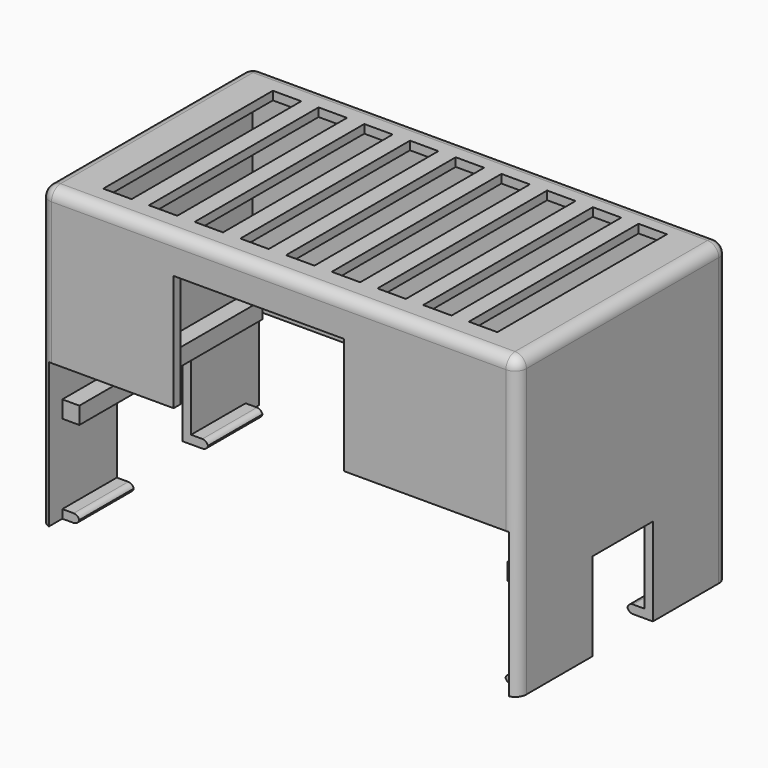
from build123d import *

# Parameters (mm, degrees)
F0_W         = 84
F0_H         = 46.33
F1_DEPTH     = 37
F2_T         = -1.5
F4_W         = 81
F4_H         = 10
F5_DEPTH     = 1.5
F6_W         = 30
F6_H         = 20.5
F7_DEPTH     = 1.5
F9_DEPTH     = 15.5
F10_W        = 40.33
F10_H        = 3
F11_DEPTH    = 3
F12_W        = 39.33
F12_H        = 3
F13_DEPTH    = 3
F14_W        = 1.5
F14_H        = 13.33
F15_DEPTH    = 15.5
F16_W        = 1.5
F16_H        = 16.33
F17_DEPTH    = 15.5
F18_W        = 12
F18_H        = 1.5
F19_DEPTH    = 3
F20_W        = 13.5
F20_H        = 1.5
F21_DEPTH    = 3
F22_W        = 5
F22_H        = 37.33
F23_DEPTH    = 1.5
F24_R        = 2
F25_T1_DEPTH = 17
F25_T3_DEPTH = 17
F25_T5_DEPTH = 18.5
F25_T7_DEPTH = 18.5


# Not quite as in the source:
# - a fillet or chamfer that OpenCascade refuses, or shapes differently, is made with other operations: its cross-section is extruded or revolved along the edge and cut away or added


with BuildPart() as f1:
    # F0 (on Top) → F1 (new body)
    with BuildSketch(Plane.XY):
        with Locations((42, 23.165)):
            Rectangle(F0_W, F0_H)
    extrude(amount=-F1_DEPTH)

    # F2
    f2_openings = [f1.faces().sort_by_distance(p)[0] for p in [
        (42, 23.165, -37),
    ]]
    offset(amount=F2_T, openings=f2_openings)

    # F4 (on face) → F5 (cut, through all)
    with BuildSketch(Plane.XZ):
        with Locations((42, -32)):
            Rectangle(F4_W, F4_H)
    extrude(amount=-F5_DEPTH, mode=Mode.SUBTRACT)

    # F6 (on face) → F7 (cut, through all)
    with BuildSketch(Plane.XZ):
        with Locations((38.5, -16.75)):
            Rectangle(F6_W, F6_H)
    extrude(amount=-F7_DEPTH, mode=Mode.SUBTRACT)

    # F8 (on face) → F9 (join)
    with BuildSketch(Plane(origin=(0, 0, -37), x_dir=(1, 0, 0), z_dir=(0, 0, -1))):
        Polygon((0, 0), (0, -46.33), (1.5, -46.33), (1.5, -44.83), (1.5, 0), align=None)
        Polygon((82.5, -44.83), (82.5, -46.33), (84, -46.33), (84, 0), (82.5, 0), align=None)
    extrude(amount=F9_DEPTH)

    # F10 (on face) → F11 (join)
    with BuildSketch(Plane.YZ.offset(1.5)):
        with Locations((23.165, -35.5)):
            Rectangle(F10_W, F10_H)
    extrude(amount=F11_DEPTH)

    # F12 (on face) → F13 (join)
    with BuildSketch(Plane(origin=(82.5, 0, 0), x_dir=(0, -1, 0), z_dir=(-1, 0, 0))):
        with Locations((-23.165, -35.5)):
            Rectangle(F12_W, F12_H)
    extrude(amount=F13_DEPTH)

    # F14 (on face) → F15 (cut)
    with BuildSketch(Plane(origin=(0, 0, -52.5), x_dir=(1, 0, 0), z_dir=(0, 0, -1))):
        with Locations((83.25, -23.165)):
            Rectangle(F14_W, F14_H)
    extrude(amount=-F15_DEPTH, mode=Mode.SUBTRACT)

    # F16 (on face) → F17 (cut)
    with BuildSketch(Plane(origin=(0, 0, -52.5), x_dir=(1, 0, 0), z_dir=(0, 0, -1))):
        with Locations((0.75, -23.165)):
            Rectangle(F16_W, F16_H)
    extrude(amount=-F17_DEPTH, mode=Mode.SUBTRACT)

    # F18 (on face) → F19 (join)
    with BuildSketch(Plane.YZ.offset(1.5)):
        with Locations((37.33, -51.75)):
            Rectangle(F18_W, F18_H)
        with Locations((9, -51.75)):
            Rectangle(F18_W, F18_H)
    extrude(amount=F19_DEPTH)

    # F20 (on face) → F21 (join)
    with BuildSketch(Plane(origin=(82.5, 0, 0), x_dir=(0, -1, 0), z_dir=(-1, 0, 0))):
        with Locations((-9.75, -51.75)):
            Rectangle(F20_W, F20_H)
        with Locations((-36.58, -51.75)):
            Rectangle(F20_W, F20_H)
    extrude(amount=F21_DEPTH)

    # F22 (on face) → F23 (cut, through all)
    with BuildSketch(Plane(origin=(0, 0, -1.5), x_dir=(1, 0, 0), z_dir=(0, 0, -1))):
        with Locations((73.9982255152, -23.6415825304)):
            Rectangle(F22_W, F22_H)
        with Locations((65.9984473258, -23.5820097141)):
            Rectangle(F22_W, F22_H)
        with Locations((49.998890947, -23.4628640815)):
            Rectangle(F22_W, F22_H)
        with Locations((41.9991127576, -23.4032912652)):
            Rectangle(F22_W, F22_H)
        with Locations((33.9993345682, -23.3437184489)):
            Rectangle(F22_W, F22_H)
        with Locations((25.9995563788, -23.2841456326)):
            Rectangle(F22_W, F22_H)
        with Locations((17.9997781894, -23.2245728163)):
            Rectangle(F22_W, F22_H)
        with Locations((10, -23.165)):
            Rectangle(F22_W, F22_H)
        with Locations((57.9986691364, -23.5224368978)):
            Rectangle(F22_W, F22_H)
    extrude(amount=-F23_DEPTH, mode=Mode.SUBTRACT)

    # F24
    f24_edges = [f1.edges().sort_by_distance(p)[0] for p in [
        (42, 0, 0),
        (84, 23.165, 0),
        (84, 0, -26.25),
        (84, 46.33, -26.25),
        (42, 46.33, 0),
        (0, 46.33, -26.25),
        (0, 23.165, 0),
        (0, 0, -26.25),
    ]]
    fillet(f24_edges, radius=F24_R)

    # F25: fillet of radius 1 on 8 edges, made by hand

    # F25_s2 → F25_t1 (cut)
    with BuildSketch(Plane.XZ.offset(-17.5)):
        with BuildLine():
            ThreePointArc((3.5, -52.5), (4.2071067812, -52.2071067812), (4.5, -51.5))
            Line((4.5, -51.5), (4.5, -52.5))
            Line((4.5, -52.5), (3.5, -52.5))
        make_face()
        with BuildLine():
            ThreePointArc((4.5, -52), (4.2071067812, -51.2928932188), (3.5, -51))
            Line((3.5, -51), (4.5, -51))
            Line((4.5, -51), (4.5, -52))
        make_face()
    extrude(amount=F25_T1_DEPTH, mode=Mode.SUBTRACT)

    # F25_s4 → F25_t3 (cut)
    with BuildSketch(Plane.XZ.offset(-45.83)):
        with BuildLine():
            ThreePointArc((3.5, -52.5), (4.2071067812, -52.2071067812), (4.5, -51.5))
            Line((4.5, -51.5), (4.5, -52.5))
            Line((4.5, -52.5), (3.5, -52.5))
        make_face()
        with BuildLine():
            ThreePointArc((3.5, -51), (4.2071067812, -51.2928932188), (4.5, -52))
            Line((4.5, -52), (4.5, -51))
            Line((4.5, -51), (3.5, -51))
        make_face()
    extrude(amount=F25_T3_DEPTH, mode=Mode.SUBTRACT)

    # F25_s6 → F25_t5 (cut)
    with BuildSketch(Plane.XZ.offset(-19)):
        with BuildLine():
            ThreePointArc((80.5, -51), (79.7928932188, -51.2928932188), (79.5, -52))
            Line((79.5, -52), (79.5, -51))
            Line((79.5, -51), (80.5, -51))
        make_face()
        with BuildLine():
            ThreePointArc((80.5, -52.5), (79.7928932188, -52.2071067812), (79.5, -51.5))
            Line((79.5, -51.5), (79.5, -52.5))
            Line((79.5, -52.5), (80.5, -52.5))
        make_face()
    extrude(amount=F25_T5_DEPTH, mode=Mode.SUBTRACT)

    # F25_s8 → F25_t7 (cut)
    with BuildSketch(Plane.XZ.offset(-45.83)):
        with BuildLine():
            ThreePointArc((80.5, -52.5), (79.7928932188, -52.2071067812), (79.5, -51.5))
            Line((79.5, -51.5), (79.5, -52.5))
            Line((79.5, -52.5), (80.5, -52.5))
        make_face()
        with BuildLine():
            ThreePointArc((80.5, -51), (79.7928932188, -51.2928932188), (79.5, -52))
            Line((79.5, -52), (79.5, -51))
            Line((79.5, -51), (80.5, -51))
        make_face()
    extrude(amount=F25_T7_DEPTH, mode=Mode.SUBTRACT)


solid = f1.part
